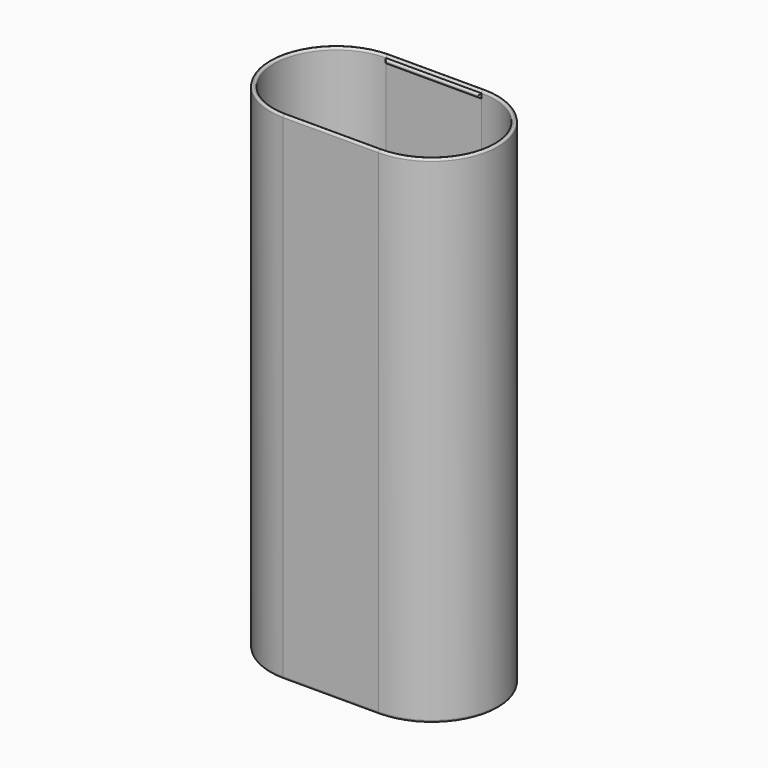
from build123d import *

# Parameters (mm, degrees)
F0_W     = 14.5
F0_H     = 7.5
F1_DEPTH = 0.8
F2_DEPTH = 93.6
F3_R     = 0.39999
F4_R     = 0.4
F5_W     = 18
F5_H     = 0.8
F6_W     = 18
F6_H     = 0.8
F7_DEPTH = 0.4
F8_R     = 0.39999


# Not quite as in the source:
# - a fillet or chamfer is up to 0.001 mm smaller than in the source, because OpenCascade refuses the exact size
# - a feature names something its author has since deleted; it is built from what else it names


with BuildPart() as f1:
    # F0 (on Top) → F1 (new body)
    with BuildSketch(Plane.XY):
        with BuildLine():
            Line((9, 12.55), (-9, 12.55))
            ThreePointArc((-9, 12.55), (-21.55, 0), (-9, -12.55))
            Line((-9, -12.55), (9, -12.55))
            ThreePointArc((9, -12.55), (21.55, 0), (9, 12.55))
        make_face()
        with BuildLine():
            ThreePointArc((-9, -11.75), (-20.75, 0), (-9, 11.75))
            Line((-9, 11.75), (9, 11.75))
            ThreePointArc((9, 11.75), (20.75, 0), (9, -11.75))
            Line((9, -11.75), (-9, -11.75))
        make_face(mode=Mode.SUBTRACT)
        with BuildLine():
            Line((9, 11.75), (-9, 11.75))
            ThreePointArc((-9, 11.75), (-20.75, 0), (-9, -11.75))
            Line((-9, -11.75), (9, -11.75))
            ThreePointArc((9, -11.75), (20.75, 0), (9, 11.75))
        make_face()
        with Locations((-7.25, 0)):
            Rectangle(F0_W, F0_H, mode=Mode.SUBTRACT)
    extrude(amount=F1_DEPTH)

    # F0 (on Top) → F2 (join)
    with BuildSketch(Plane.XY):
        with BuildLine():
            Line((9, 12.55), (-9, 12.55))
            ThreePointArc((-9, 12.55), (-21.55, 0), (-9, -12.55))
            Line((-9, -12.55), (9, -12.55))
            ThreePointArc((9, -12.55), (21.55, 0), (9, 12.55))
        make_face()
        with BuildLine():
            ThreePointArc((-9, -11.75), (-20.75, 0), (-9, 11.75))
            Line((-9, 11.75), (9, 11.75))
            ThreePointArc((9, 11.75), (20.75, 0), (9, -11.75))
            Line((9, -11.75), (-9, -11.75))
        make_face(mode=Mode.SUBTRACT)
    extrude(amount=F2_DEPTH)

    # F3 (radius 0.4 in the source; OpenCascade refuses exactly that, so slightly less here)
    f3_edges = [f1.edges().sort_by_distance(p)[0] for p in [
        (0, -12.55, 93.6),
        (0, -11.75, 93.6),
        (0, -12.55, 0),
        (-7.25, 3.75, 0),
        (-7.25, 3.75, 0.8),
        (-14.5, 0, 0),
        (-14.5, 0, 0.8),
        (-7.25, -3.75, 0),
        (-7.25, -3.75, 0.8),
        (0, 0, 0),
        (0, 0, 0.8),
    ]]
    fillet(f3_edges, radius=F3_R)

    # F4
    f4_edges = [f1.edges().sort_by_distance(p)[0] for p in [
        (0, 11.75, 0.8),
    ]]
    fillet(f4_edges, radius=F4_R)

    # F5 (on face) + F6 (on face) → F7 (join, symmetric)
    with BuildSketch(Plane.XZ.offset(-11.75)):
        with Locations((0, 92.8)):
            Rectangle(F5_W, F5_H)
    with BuildSketch(Plane(origin=(0, -11.75, 0), x_dir=(-1, 0, 0), z_dir=(0, 1, 0))):
        with Locations((0, 92.8)):
            Rectangle(F6_W, F6_H)
    extrude(amount=F7_DEPTH, both=True, dir=(0, -1, 0))

    # F8 (radius 0.4 in the source; OpenCascade refuses exactly that, so slightly less here)
    f8_edges = [f1.edges().sort_by_distance(p)[0] for p in [
        (0, 11.35, 93.2),
        (0, 11.35, 92.4),
        (-9, 11.35, 92.8),
        (9, 11.35, 92.8),
        (0, -11.35, 93.2),
        (0, -11.35, 92.4),
        (9, -11.35, 92.8),
        (-9, -11.35, 92.8),
    ]]
    fillet(f8_edges, radius=F8_R)


solid = f1.part
